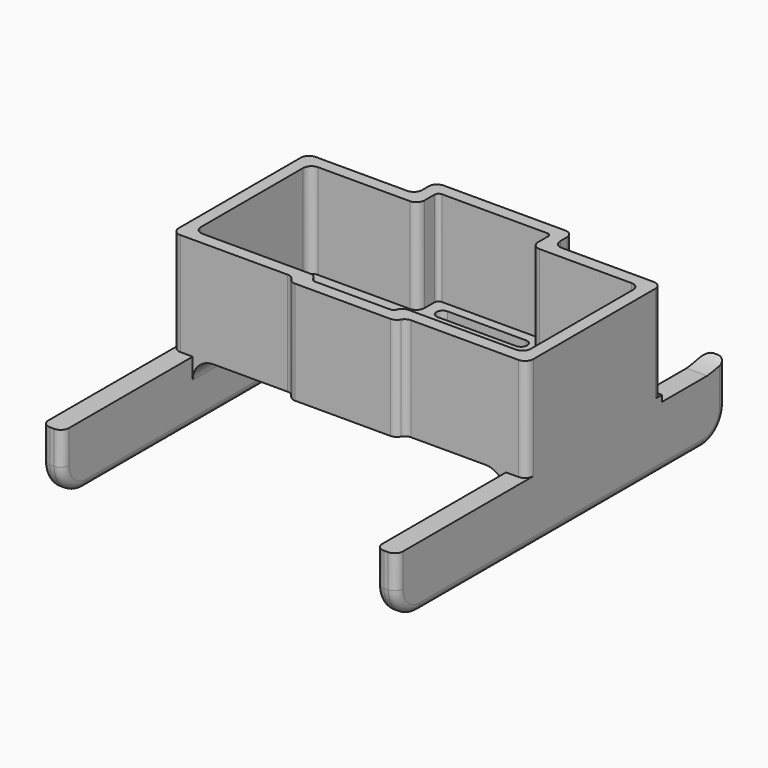
from build123d import *

# Parameters (mm, degrees)
F1_DEPTH      = 2
F2_DEPTH      = 25
F3_W          = 5
F3_H          = 60
F4_DEPTH      = 15
F3_H_2        = 40
F5_DEPTH      = 15
F5_DEPTH_BACK = 1.5
F6_R          = 7
F8_DEPTH      = 86.001
F7_W          = 6.048347801
F7_H          = 1.5
F9_DEPTH      = 5.1
F10_W         = 6
F10_H         = 1.5
F11_DEPTH     = 5.1
F12_T1_DEPTH  = 41
F12_T3_DEPTH  = 40.980202511
F12_T8_DEPTH  = 53.480202511
F13_R         = 2


# Not quite as in the source:
# - a fillet or chamfer that OpenCascade refuses, or shapes differently, is made with other operations: its cross-section is extruded or revolved along the edge and cut away or added


with BuildPart() as f1:
    # F0 (on Top) → F1 (new body)
    with BuildSketch(Plane.XY):
        with BuildLine():
            ThreePointArc((40, 15.5), (39.4142135624, 16.9142135624), (38, 17.5))
            Line((38, 17.5), (15.75, 17.5))
            ThreePointArc((15.75, 17.5), (14.3357864376, 18.0857864376), (13.75, 19.5))
            Line((13.75, 19.5), (13.75, 22.5))
            ThreePointArc((13.75, 22.5), (13.4571067812, 23.2071067812), (12.75, 23.5))
            Line((12.75, 23.5), (-12.75, 23.5))
            ThreePointArc((-12.75, 23.5), (-13.4571067812, 23.2071067812), (-13.75, 22.5))
            Line((-13.75, 22.5), (-13.75, 19.5))
            ThreePointArc((-13.75, 19.5), (-14.3357864376, 18.0857864376), (-15.75, 17.5))
            Line((-15.75, 17.5), (-38, 17.5))
            ThreePointArc((-38, 17.5), (-39.4142135624, 16.9142135624), (-40, 15.5))
            Line((-40, 15.5), (-40, -15.5))
            ThreePointArc((-40, -15.5), (-39.4142135624, -16.9142135624), (-38, -17.5))
            Line((-38, -17.5), (-12, -17.5))
            ThreePointArc((-12, -17.5), (-11.4705903261, -17.5713410366), (-10.978949287, -17.7802746029))
            ThreePointArc((-10.978949287, -17.7802746029), (-10.4680840625, -16.8849116385), (-9.5, -16.5306922667))
            Line((-9.5, -16.5306922667), (0, -16.5306922667))
            Line((0, -16.5306922667), (9.5, -16.5306922667))
            ThreePointArc((9.5, -16.5306922667), (10.4680840625, -16.8849116385), (10.978949287, -17.7802746029))
            ThreePointArc((10.978949287, -17.7802746029), (11.4705903261, -17.5713410366), (12, -17.5))
            Line((12, -17.5), (38, -17.5))
            ThreePointArc((38, -17.5), (39.4142135624, -16.9142135624), (40, -15.5))
            Line((40, -15.5), (40, 15.5))
        make_face()
        with BuildLine():
            ThreePointArc((-9.5, 18.1578074247), (-11, 19.6578074247), (-9.5, 21.1578074247))
            Line((-9.5, 21.1578074247), (0, 21.1578074247))
            Line((0, 21.1578074247), (9.5, 21.1578074247))
            ThreePointArc((9.5, 21.1578074247), (11, 19.6578074247), (9.5, 18.1578074247))
            Line((9.5, 18.1578074247), (0, 18.1578074247))
            Line((0, 18.1578074247), (-9.5, 18.1578074247))
        make_face(mode=Mode.SUBTRACT)
    extrude(amount=F1_DEPTH)

    # F0 (on Top) → F2 (join)
    with BuildSketch(Plane.XY):
        with BuildLine():
            ThreePointArc((43, 18.5), (42.4142135624, 19.9142135624), (41, 20.5))
            Line((41, 20.5), (18.75, 20.5))
            ThreePointArc((18.75, 20.5), (17.3357864376, 21.0857864376), (16.75, 22.5))
            Line((16.75, 22.5), (16.75, 24.5))
            ThreePointArc((16.75, 24.5), (16.1642135624, 25.9142135624), (14.75, 26.5))
            Line((14.75, 26.5), (-14.75, 26.5))
            ThreePointArc((-14.75, 26.5), (-16.1642135624, 25.9142135624), (-16.75, 24.5))
            Line((-16.75, 24.5), (-16.75, 22.5))
            ThreePointArc((-16.75, 22.5), (-17.3357864376, 21.0857864376), (-18.75, 20.5))
            Line((-18.75, 20.5), (-41, 20.5))
            ThreePointArc((-41, 20.5), (-42.4142135624, 19.9142135624), (-43, 18.5))
            Line((-43, 18.5), (-43, -18.5))
            ThreePointArc((-43, -18.5), (-42.4142135624, -19.9142135624), (-41, -20.5))
            Line((-41, -20.5), (-15, -20.5))
            ThreePointArc((-15, -20.5), (-14, -20.7679491924), (-13.2679491924, -21.5))
            ThreePointArc((-13.2679491924, -21.5), (-12.5358983849, -22.2320508076), (-11.5358983849, -22.5))
            Line((-11.5358983849, -22.5), (11.5358983849, -22.5))
            ThreePointArc((11.5358983849, -22.5), (12.5358983849, -22.2320508076), (13.2679491924, -21.5))
            ThreePointArc((13.2679491924, -21.5), (14, -20.7679491924), (15, -20.5))
            Line((15, -20.5), (41, -20.5))
            ThreePointArc((41, -20.5), (42.4142135624, -19.9142135624), (43, -18.5))
            Line((43, -18.5), (43, 18.5))
        make_face()
        with BuildLine():
            Line((15.75, 17.5), (38, 17.5))
            ThreePointArc((38, 17.5), (39.4142135624, 16.9142135624), (40, 15.5))
            Line((40, 15.5), (40, -15.5))
            ThreePointArc((40, -15.5), (39.4142135624, -16.9142135624), (38, -17.5))
            Line((38, -17.5), (12, -17.5))
            ThreePointArc((12, -17.5), (11.4705903261, -17.5713410366), (10.978949287, -17.7802746029))
            ThreePointArc((10.978949287, -17.7802746029), (10.4542270396, -18.2309113684), (10.1143819168, -18.8333333333))
            ThreePointArc((10.1143819168, -18.8333333333), (9.7489231444, -19.3164965809), (9.1715728753, -19.5))
            Line((9.1715728753, -19.5), (0, -19.5))
            Line((0, -19.5), (-9.1715728753, -19.5))
            Line((-9.1715728753, -19.5), (-9.1981146163, -19.5))
            ThreePointArc((-9.1981146163, -19.5), (-9.1973546351, -19.4998436487), (-9.1965947349, -19.4996869043))
            ThreePointArc((-9.1965947349, -19.4996869043), (-9.7590938823, -19.3092089139), (-10.1143819168, -18.8333333333))
            ThreePointArc((-10.1143819168, -18.8333333333), (-10.4542270396, -18.2309113684), (-10.978949287, -17.7802746029))
            ThreePointArc((-10.978949287, -17.7802746029), (-11.4705903261, -17.5713410366), (-12, -17.5))
            Line((-12, -17.5), (-38, -17.5))
            ThreePointArc((-38, -17.5), (-39.4142135624, -16.9142135624), (-40, -15.5))
            Line((-40, -15.5), (-40, 15.5))
            ThreePointArc((-40, 15.5), (-39.4142135624, 16.9142135624), (-38, 17.5))
            Line((-38, 17.5), (-15.75, 17.5))
            ThreePointArc((-15.75, 17.5), (-14.3357864376, 18.0857864376), (-13.75, 19.5))
            Line((-13.75, 19.5), (-13.75, 22.5))
            ThreePointArc((-13.75, 22.5), (-13.4571067812, 23.2071067812), (-12.75, 23.5))
            Line((-12.75, 23.5), (12.75, 23.5))
            ThreePointArc((12.75, 23.5), (13.4571067812, 23.2071067812), (13.75, 22.5))
            Line((13.75, 22.5), (13.75, 19.5))
            ThreePointArc((13.75, 19.5), (14.3357864376, 18.0857864376), (15.75, 17.5))
        make_face(mode=Mode.SUBTRACT)
    extrude(amount=F2_DEPTH)

    # F3 (on Top) → F4 (join)
    with BuildSketch(Plane.XY):
        with Locations((-40.5, -30)):
            Rectangle(F3_W, F3_H)
        with Locations((40.5, -30)):
            Rectangle(F3_W, F3_H)
    extrude(amount=-F4_DEPTH)

    # F3 (on Top) → F5 (join, two sides)
    with BuildSketch(Plane.XY) as f5_sk:
        with Locations((-40.5, 20)):
            Rectangle(F3_W, F3_H_2)
        with Locations((40.5, 20)):
            Rectangle(F3_W, F3_H_2)
    extrude(amount=-F5_DEPTH)
    extrude(f5_sk.sketch, amount=F5_DEPTH_BACK)

    # F6
    f6_edges = [f1.edges().sort_by_distance(p)[0] for p in [
        (40.5, 40, -15),
        (-40.5, 40, -15),
        (-40.5, -60, -15),
        (40.5, -60, -15),
    ]]
    fillet(f6_edges, radius=F6_R)

    # F7 (on face) → F8 (cut, through all)
    with BuildSketch(Plane(origin=(-43, 0, 0), x_dir=(0, -1, 0), z_dir=(-1, 0, 0))):
        with BuildLine():
            Line((-26.5285503119, 1.5), (-40, 1.5))
            add(Edge.make_bspline(
                [(-40, 1.5), (-39.5081001265, 1.219408998), (-38.2821576057, 0.5201031862), (-35.7543121769, 0.1947861269), (-34.240745008, 0)],
                knots=[0, 0, 0, 0, 0.4012421995, 1, 1, 1, 1], degree=3))
            Line((-34.240745008, 0), (-26.5285503119, 0))
            Line((-26.5285503119, 0), (-26.5285503119, 1.5))
        make_face()
    extrude(amount=-F8_DEPTH, mode=Mode.SUBTRACT)

    # F7 (on face) → F9 (cut)
    with BuildSketch(Plane(origin=(-43, 0, 0), x_dir=(0, -1, 0), z_dir=(-1, 0, 0))):
        with Locations((-23.5043764114, 0.75)):
            Rectangle(F7_W, F7_H)
    extrude(amount=-F9_DEPTH, mode=Mode.SUBTRACT)

    # F10 (on face) → F11 (cut)
    with BuildSketch(Plane.YZ.offset(43)):
        with Locations((23.5285503119, 0.75)):
            Rectangle(F10_W, F10_H)
    extrude(amount=-F11_DEPTH, mode=Mode.SUBTRACT)

    # F12: fillet of radius 5 on 2 edges, made by hand

    # F12_s2 → F12_t1 (join)
    with BuildSketch(Plane.XZ.offset(-20.5)):
        with BuildLine():
            ThreePointArc((38, -5), (36.5355339059, -1.4644660941), (33, 0))
            Line((33, 0), (38, 0))
            Line((38, 0), (38, -5))
        make_face()
    extrude(amount=F12_T1_DEPTH)

    # F12_s4 → F12_t3 (join)
    with BuildSketch(Plane.XZ.offset(-20.480202511)):
        with BuildLine():
            ThreePointArc((-38, -5), (-36.5355339059, -1.4644660941), (-33, 0))
            Line((-33, 0), (-38, 0))
            Line((-38, 0), (-38, -5))
        make_face()
    extrude(amount=F12_T3_DEPTH)


with BuildPart() as f12_tool6:
    # F12_s7 → F12_t8 (new body)
    with BuildSketch(Plane.XZ.offset(20.5)):
        with BuildLine():
            ThreePointArc((-38, -5), (-36.5355339059, -1.4644660941), (-33, 0))
            Line((-33, 0), (-38, 0))
            Line((-38, 0), (-38, -5))
        make_face()
    extrude(amount=-F12_T8_DEPTH)

    split(bisect_by=Plane.XZ.offset(-20.5), keep=Keep.TOP)

    split(bisect_by=Plane.YZ.offset(-37.9), keep=Keep.TOP)


with BuildPart() as f1_1:
    add(f1.part)

    # F12_t5: union F12_tool6
    add(f12_tool6.part)

    # F13
    f13_edges = [f1_1.edges().sort_by_distance(p)[0] for p in [
        (-38, 40, -3.25),
        (-43, 40, -3.25),
        (38, 40, -3.25),
        (43, 40, -3.25),
        (43, 37.949747, -12.949747),
        (43, -10, -15),
        (43, -57.949747, -12.949747),
        (43, -60, -4),
        (38, -57.949747, -12.949747),
        (38, -60, -4),
        (38, 37.949747, -12.949747),
        (38, -10, -15),
        (-38, -60, -4),
        (-38, 37.949747, -12.949747),
        (-38, -10, -15),
        (-38, -57.949747, -12.949747),
        (-43, -57.949747, -12.949747),
        (-43, -10, -15),
        (-43, 37.949747, -12.949747),
        (-43, -60, -4),
    ]]
    fillet(f13_edges, radius=F13_R)


solid = f1_1.part
